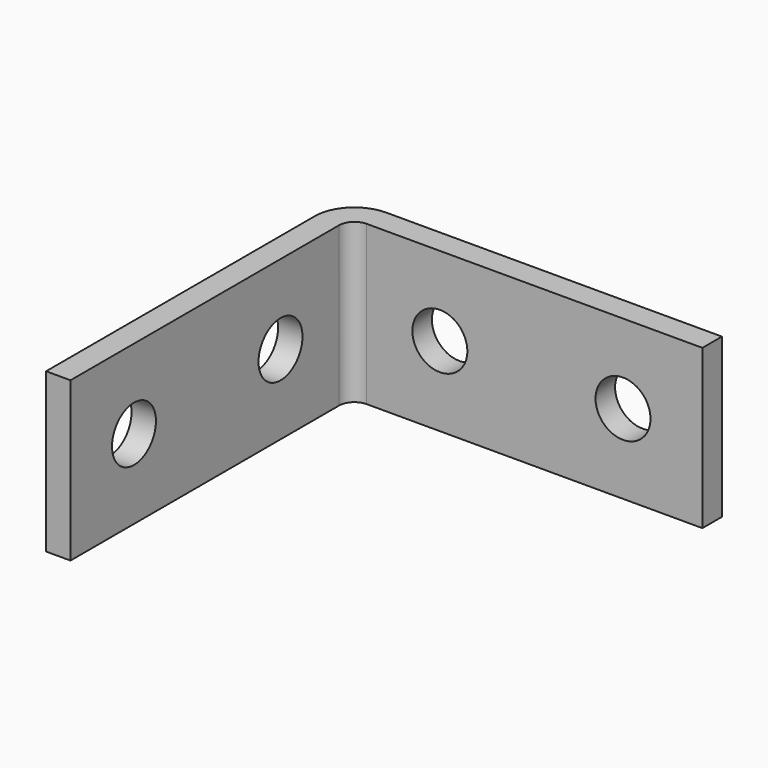
from build123d import *

# Parameters (mm, degrees)
F1_DEPTH = 41.275
F4_D     = 14.2875
F7_D     = 14.2875


# Not quite as in the source:
# - a length typed as a fraction of an inch, garbled in the dataset ("3 / 203.2 mm" for 3/8 in), is restored


with BuildPart() as f1:
    # F0 (on Top) → F1 (new body)
    with BuildSketch(Plane.XY):
        with BuildLine():
            ThreePointArc((10.31875, 97.63125), (3.0222919016, 94.6089580984), (0, 87.3125))
            Line((0, 87.3125), (0, 0))
            Line((0, 0), (6.35, 0))
            Line((6.35, 0), (6.35, 87.3125))
            ThreePointArc((6.35, 87.3125), (7.5124199622, 90.1188300378), (10.31875, 91.28125))
            Line((10.31875, 91.28125), (97.63125, 91.28125))
            Line((97.63125, 91.28125), (97.63125, 97.63125))
            Line((97.63125, 97.63125), (10.31875, 97.63125))
        make_face()
    extrude(amount=F1_DEPTH)

    # F4 (through all)
    with Locations(Plane.YZ.offset(6.35)):
        with Locations((20.6375, 20.6375), (68.2625, 20.6375)):
            Hole(F4_D / 2)

    # F7 (through all)
    with Locations(Plane.XZ.offset(-91.28125)):
        with Locations((29.36875, 20.6375), (76.99375, 20.6375)):
            Hole(F7_D / 2)


solid = f1.part
